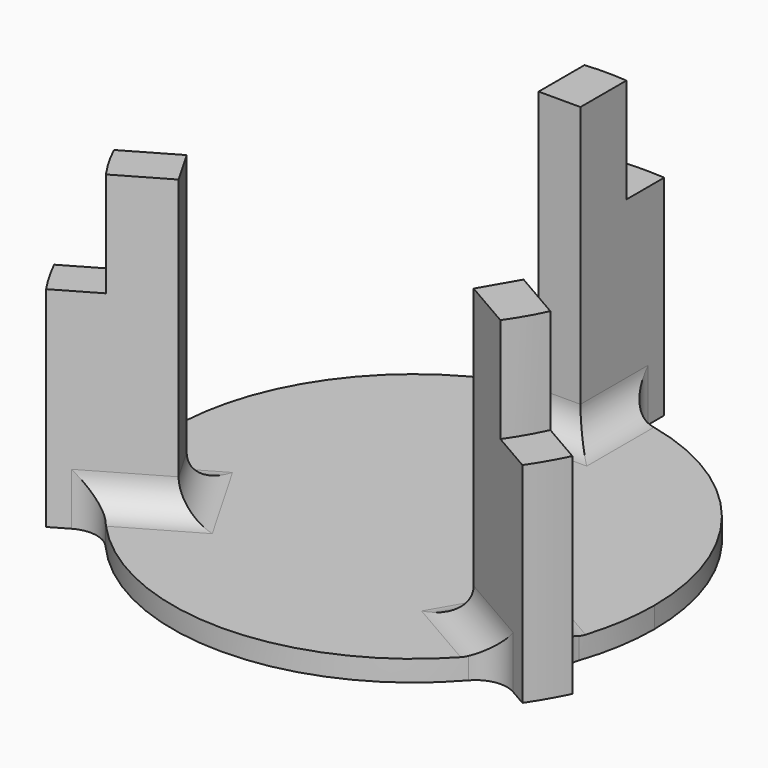
from build123d import *

# Parameters (mm, degrees)
F5_DEPTH = 30
F6_DEPTH = 20
F0_COUNT = 3
F1_DEPTH = 2
F2_R     = 3


# Not quite as in the source:
# - a feature names something its author has since deleted; it is built from what else it names


with BuildPart() as f5:
    # F4 (on Top) → F5 (new body)
    with BuildSketch(Plane.XY):
        with BuildLine():
            ThreePointArc((2, 22.9128784748), (0, 23), (-2, 22.9128784748))
            Line((-2, 22.9128784748), (-2, 17.4271763038))
            Line((-2, 17.4271763038), (2, 17.4271763038))
            Line((2, 17.4271763038), (2, 22.9128784748))
        make_face()
    extrude(amount=F5_DEPTH)

    # F4 (on Top) → F6 (join)
    with BuildSketch(Plane.XY):
        with BuildLine():
            Line((2, 24.4271763038), (2, 27.4271763038))
            Line((2, 27.4271763038), (-2, 27.4271763038))
            Line((-2, 27.4271763038), (-2, 22.9128784748))
            ThreePointArc((-2, 22.9128784748), (0, 23), (2, 22.9128784748))
            Line((2, 22.9128784748), (2, 24.4271763038))
        make_face()
        with BuildLine():
            Line((-2, 27.4271763038), (2, 27.4271763038))
            ThreePointArc((2, 27.4271763038), (0, 27.5), (-2, 27.4271763038))
        make_face()
    extrude(amount=F6_DEPTH)


with BuildPart() as f0_1:
    # F0: instance of F5
    add(f5.part.rotate(Axis((0, 0, 0), (0, 0, 1)), 1 * 360 / F0_COUNT))


with BuildPart() as f0_2:
    # F0: instance of F5
    add(f5.part.rotate(Axis((0, 0, 0), (0, 0, 1)), 2 * 360 / F0_COUNT))


with BuildPart() as f5_1:
    add(f5.part)

    add(f0_1.part)  # F1 merges F0_1

    add(f0_2.part)  # F1 merges F0_2
    # F4 (on Top) → F1 (join)
    with BuildSketch(Plane.XY):
        with BuildLine():
            ThreePointArc((2, 22.9128784748), (0, 23), (-2, 22.9128784748))
            Line((-2, 22.9128784748), (-2, 17.4271763038))
            Line((-2, 17.4271763038), (2, 17.4271763038))
            Line((2, 17.4271763038), (2, 22.9128784748))
        make_face()
        with BuildLine():
            Line((-2, 17.4271763038), (-2, 22.9128784748))
            ThreePointArc((-2, 22.9128784748), (-15.5402702679, -16.9558249578), (23, 0))
            ThreePointArc((23, 0), (16.9558249578, 15.5402702679), (2, 22.9128784748))
            Line((2, 22.9128784748), (2, 17.4271763038))
            Line((2, 17.4271763038), (-2, 17.4271763038))
        make_face()
    extrude(amount=F1_DEPTH)

    # F2
    f2_edges = [f5_1.edges().sort_by_distance(p)[0] for p in [
        (-2, 20.170027, 2),
        (0, 17.427176, 2),
        (2, 20.170027, 2),
        (16.467756, -11.817065, 2),
        (15.092377, -8.713588, 2),
        (18.467756, -8.352963, 2),
        (-18.467756, -8.352963, 2),
        (-15.092377, -8.713588, 2),
        (-16.467756, -11.817065, 2),
        (-2, 22.912878, 1),
        (-20.843135, -9.724388, 1),
        (2, 22.912878, 1),
        (20.843135, -9.724388, 1),
        (18.843135, -13.18849, 1),
        (-18.843135, -13.18849, 1),
    ]]
    fillet(f2_edges, radius=F2_R)


solid = f5_1.part
